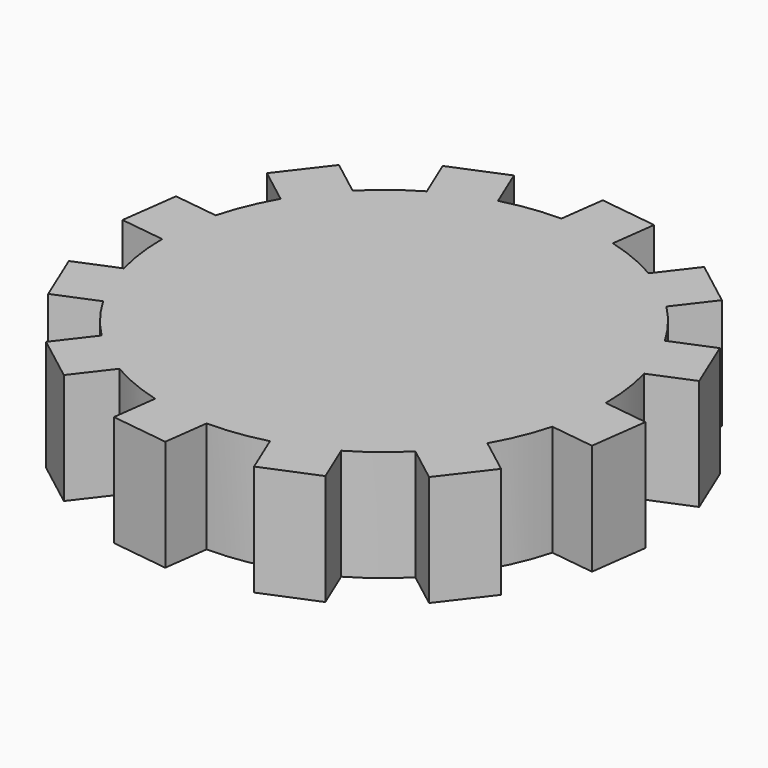
from build123d import *

# Parameters (mm, degrees)
F1_DEPTH = 3.175
F2_COUNT = 12


# Not quite as in the source:
# - a length typed as a fraction of an inch, garbled in the dataset ("3 / 203.2 mm" for 3/8 in), is restored


with BuildPart() as f1:
    # F0 (on Top) → F1 (new body)
    with BuildSketch(Plane.XY):
        with BuildLine():
            ThreePointArc((0, 6.35), (-4.4901280605, -4.4901280605), (6.35, 0))
            ThreePointArc((6.35, 0), (5.0377937108, 3.8656350742), (1.6435009364, 6.1336289969))
            ThreePointArc((1.6435009364, 6.1336289969), (0.8288413206, 6.2956748697), (0, 6.35))
        make_face()
        with BuildLine():
            ThreePointArc((0, 6.35), (0.8288413206, 6.2956748697), (1.6435009364, 6.1336289969))
            Line((1.6435009364, 6.1336289969), (1.8104587787, 7.4017997143))
            Line((1.8104587787, 7.4017997143), (0.1669578423, 7.6181707174))
            Line((0.1669578423, 7.6181707174), (0, 6.35))
        make_face()
    extrude(amount=F1_DEPTH)

    # F2: F1 ×12 about axis
    f2_axis = Axis((0, 0, 0), (0, 0, -1))


with BuildPart() as f1_1:
    add(f1.part)
    for i in range(1, F2_COUNT):
        add(f1.part.rotate(f2_axis, i * 360 / F2_COUNT))


solid = f1_1.part
